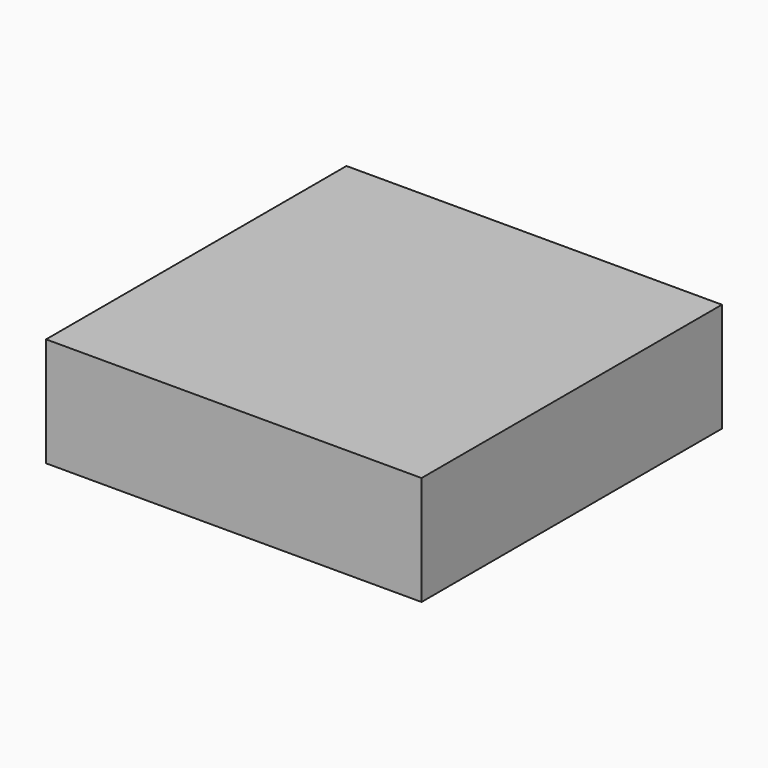
from build123d import *

# Parameters (mm, degrees)
F0_W     = 172
F0_H     = 172
F1_DEPTH = 50
F2_W     = 162
F2_H     = 162
F2_W_2   = 122
F2_H_2   = 122
F3_DEPTH = 45
F4_T     = -2.5
F5_R     = 5
F6_DEPTH = 9.5


# Not quite as in the source:
# - a shell that OpenCascade refuses in one call is made with other operations: the cavity is built on its own and cut out


with BuildPart() as f1:
    # F0 (on Top) → F1 (new body)
    with BuildSketch(Plane.XY):
        Rectangle(F0_W, F0_H)
    extrude(amount=F1_DEPTH)

    # F2 (on Top) → F3 (cut)
    with BuildSketch(Plane.XY):
        Rectangle(F2_W, F2_H)
        Rectangle(F2_W_2, F2_H_2, mode=Mode.SUBTRACT)
    extrude(amount=F3_DEPTH, mode=Mode.SUBTRACT)

    # F4: a shell. OpenCascade refuses it in one call, so the cavity is built on its own and cut out:
    # the body offset inwards by the wall thickness, plus a prism from it out through each open face.
    f4_core = offset(f1.part, amount=F4_T, kind=Kind.INTERSECTION, mode=Mode.PRIVATE)
    f4_exits = [f4_core.faces().sort_by_distance(p)[0] for p in [
        (0, 0, 2.5),
    ]]
    add(f4_core, mode=Mode.SUBTRACT)
    extrude(f4_exits, amount=-F4_T, mode=Mode.SUBTRACT)

    # F5 (on face) → F6 (cut)
    with BuildSketch(Plane(origin=(0, 86, 0), x_dir=(-1, 0, 0), z_dir=(0, 1, 0))):
        with Locations((42.7398793399, 25)):
            Circle(F5_R)
        with Locations((-42.7398793399, 25)):
            Circle(F5_R)
    extrude(amount=-F6_DEPTH, mode=Mode.SUBTRACT)


solid = f1.part
